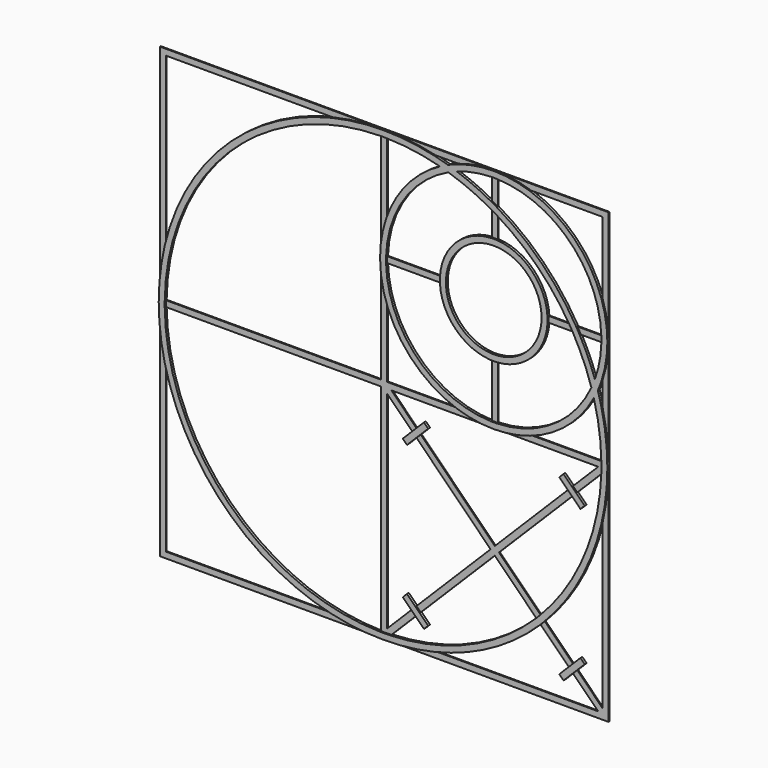
from build123d import *

# Parameters (mm, degrees)
F1_DEPTH = 0.8
F0_R     = 16
F2_DEPTH = 0.35


# Not quite as in the source:
# - a feature names something its author has since deleted; it is built from what else it names


with BuildPart() as f1:
    # F0 (on Front) → F1 (new body)
    with BuildSketch(Plane.XZ):
        with BuildLine():
            ThreePointArc((17.2103480163, 73.0397421615), (8.6659515201, 74.5380642902), (0.0056974823, 75.0397421615))
            ThreePointArc((0.0056974823, 75.0397421615), (-8.6545565556, 74.5380642902), (-17.1989530518, 73.0397421615))
            Line((-17.1989530518, 73.0397421615), (-0.9943025177, 73.0397421615))
            Line((-0.9943025177, 73.0397421615), (-0.9943025177, 73.032892525))
            ThreePointArc((-0.9943025177, 73.032892525), (0.0056974823, 73.0397421615), (1.0056974823, 73.032892525))
            Line((1.0056974823, 73.032892525), (1.0056974823, 73.0397421615))
            Line((1.0056974823, 73.0397421615), (17.2103480163, 73.0397421615))
        make_face()
        with BuildLine():
            ThreePointArc((-72.9943025177, 17.2443926956), (-74.4926246489, 8.6999961786), (-74.9943025177, 0.0397421197))
            ThreePointArc((-74.9943025177, 0.0397421197), (-74.4926246441, -8.6205118971), (-72.9943025177, -17.1649083727))
            Line((-72.9943025177, -17.1649083727), (-72.9943025177, -0.9602578386))
            Line((-72.9943025177, -0.9602578386), (-72.9874528813, -0.9602578386))
            ThreePointArc((-72.9874528813, -0.9602578386), (-72.9943025177, 0.0397421614), (-72.9874528813, 1.0397421615))
            Line((-72.9874528813, 1.0397421615), (-72.9943025177, 1.0397421615))
            Line((-72.9943025177, 1.0397421615), (-72.9943025177, 17.2443926956))
        make_face()
        with BuildLine():
            ThreePointArc((49.1712225429, 73.0397421615), (43.1701114913, 74.536408679), (37.0056974946, 75.0397421615))
            ThreePointArc((37.0056974946, 75.0397421615), (30.8412834854, 74.536408681), (24.8401724217, 73.0397421615))
            Line((24.8401724217, 73.0397421615), (36.0056974823, 73.0397421615))
            Line((36.0056974823, 73.0397421615), (37.0056974823, 73.0397421615))
            Line((37.0056974823, 73.0397421615), (38.0056974823, 73.0397421615))
            Line((38.0056974823, 73.0397421615), (49.1712225429, 73.0397421615))
        make_face()
        with BuildLine():
            ThreePointArc((21.7169774671, 71.8284621767), (19.4730859008, 72.4691615169), (17.2103480163, 73.0397421615))
            Line((17.2103480163, 73.0397421615), (1.0056974823, 73.0397421615))
            Line((1.0056974823, 73.0397421615), (1.0056974823, 73.032892525))
            ThreePointArc((1.0056974823, 73.032892525), (10.0952946195, 72.3391199569), (19.0275514161, 70.5178882276))
            ThreePointArc((19.0275514161, 70.5178882276), (20.3593616771, 71.199652938), (21.7169774671, 71.8284621767))
        make_face()
        with BuildLine():
            Line((-0.9943025177, 73.0397421615), (-17.1989530518, 73.0397421615))
            ThreePointArc((-17.1989530518, 73.0397421615), (-53.0273111067, 53.0727507504), (-72.9943025177, 17.2443926956))
            Line((-72.9943025177, 17.2443926956), (-72.9943025177, 1.0397421615))
            Line((-72.9943025177, 1.0397421615), (-72.9874528813, 1.0397421615))
            ThreePointArc((-72.9874528813, 1.0397421615), (-51.6130975444, 51.6585371881), (-0.9943025177, 73.032892525))
            Line((-0.9943025177, 73.032892525), (-0.9943025177, 73.0397421615))
        make_face()
        with BuildLine():
            Line((-72.9943025177, -0.9602578386), (-72.9943025177, -17.1649083727))
            ThreePointArc((-72.9943025177, -17.1649083727), (-53.0273111067, -52.9932664275), (-17.1989530518, -72.9602578385))
            Line((-17.1989530518, -72.9602578385), (-0.9943025177, -72.9602578385))
            Line((-0.9943025177, -72.9602578385), (-0.9943025177, -72.9534082021))
            ThreePointArc((-0.9943025177, -72.9534082021), (-51.6130975444, -51.5790528652), (-72.9874528813, -0.9602578386))
            Line((-72.9874528813, -0.9602578386), (-72.9943025177, -0.9602578386))
        make_face()
        with BuildLine():
            ThreePointArc((73.0056974823, 49.205267222), (63.8757551674, 63.9097998465), (49.1712225429, 73.0397421615))
            Line((49.1712225429, 73.0397421615), (38.0056974823, 73.0397421615))
            Line((38.0056974823, 73.0397421615), (38.0056974823, 73.0258505923))
            ThreePointArc((38.0056974823, 73.0258505923), (62.461541605, 62.4955862842), (72.9918059132, 38.0397421615))
            Line((72.9918059132, 38.0397421615), (73.0056974823, 38.0397421615))
            Line((73.0056974823, 38.0397421615), (73.0056974823, 49.205267222))
        make_face()
        with BuildLine():
            Line((36.0056974823, 73.0397421615), (24.8401724217, 73.0397421615))
            ThreePointArc((24.8401724217, 73.0397421615), (23.265221036, 72.4685342242), (21.7169774671, 71.8284621767))
            ThreePointArc((21.7169774671, 71.8284621767), (23.204042899, 71.3618058579), (24.6810902267, 70.864349417))
            ThreePointArc((24.6810902267, 70.864349417), (30.2563040679, 72.4013836468), (36.0056974823, 73.0258505923))
            Line((36.0056974823, 73.0258505923), (36.0056974823, 73.0397421615))
        make_face()
        with BuildLine():
            ThreePointArc((24.6810902267, 70.864349417), (23.204042899, 71.3618058579), (21.7169774671, 71.8284621767))
            ThreePointArc((21.7169774671, 71.8284621767), (20.3593616771, 71.199652938), (19.0275514161, 70.5178882276))
            ThreePointArc((19.0275514161, 70.5178882276), (20.4433919435, 70.1204145691), (21.8509385418, 69.6945011019))
            ThreePointArc((21.8509385418, 69.6945011019), (23.2535693595, 70.3095328445), (24.6810902267, 70.864349417))
        make_face()
        with BuildLine():
            ThreePointArc((-17.1989530518, -72.9602578385), (-8.6545565556, -74.4585799673), (0.0056974823, -74.9602578385))
            ThreePointArc((0.0056974823, -74.9602578385), (8.6659515201, -74.4585799673), (17.2103480163, -72.9602578386))
            Line((17.2103480163, -72.9602578385), (2.4199110446, -72.9602578385))
            Line((2.4199110446, -72.9602578385), (2.3812484608, -72.9215952547))
            ThreePointArc((2.3812484608, -72.9215952547), (0.6936568848, -72.957016067), (-0.9943025177, -72.9534082021))
            Line((-0.9943025177, -72.9534082021), (-0.9943025177, -72.9602578385))
            Line((-0.9943025177, -72.9602578385), (-17.1989530518, -72.9602578385))
        make_face()
        with BuildLine():
            ThreePointArc((73.0056974823, 24.8742171009), (74.5023640008, 30.8753281585), (75.0056974823, 37.0397421615))
            ThreePointArc((75.0056974823, 37.0397421615), (74.5023640008, 43.2041561644), (73.0056974823, 49.205267222))
            Line((73.0056974823, 49.205267222), (73.0056974823, 38.0397421615))
            Line((73.0056974823, 38.0397421615), (73.0056974823, 37.0397421615))
            Line((73.0056974823, 37.0397421615), (73.0056974823, 36.0397421615))
            Line((73.0056974823, 36.0397421615), (73.0056974823, 24.8742171009))
        make_face()
        with BuildLine():
            ThreePointArc((21.8509385418, 69.6945011019), (20.4433919435, 70.1204145691), (19.0275514161, 70.5178882276))
            ThreePointArc((19.0275514161, 70.5178882276), (7.9890295703, 61.5761025942), (1.0056974823, 49.205267222))
            Line((1.0056974823, 49.205267222), (1.0056974823, 38.0397421615))
            Line((1.0056974823, 38.0397421615), (1.0195890514, 38.0397421615))
            ThreePointArc((1.0195890514, 38.0397421614), (6.9332346671, 56.8298149312), (21.8509385418, 69.6945011019))
        make_face()
        with BuildLine():
            ThreePointArc((36.0056974823, 65.8348787598), (30.4474404505, 68.5838905992), (24.6810902267, 70.864349417))
            ThreePointArc((24.6810902267, 70.864349417), (23.2535693595, 70.3095328445), (21.8509385418, 69.6945011019))
            ThreePointArc((21.8509385418, 69.6945011019), (29.0912622658, 66.9951745118), (36.0056974823, 63.5456473987))
            Line((36.0056974823, 63.5456473987), (36.0056974823, 65.8348787598))
        make_face()
        with BuildLine():
            Line((2.4199110446, -72.9602578385), (17.2103480163, -72.9602578385))
            ThreePointArc((17.2103480163, -72.9602578386), (36.078425865, -65.7155486297), (52.3268850353, -53.695658954))
            Line((52.3268850353, -53.695658954), (50.9125423033, -52.281316222))
            ThreePointArc((50.9125423033, -52.281316222), (28.6127517607, -67.1215297556), (2.4612213459, -72.9189475373))
            Line((2.4612213459, -72.9189475373), (2.4199110446, -72.9602578385))
        make_face()
        with BuildLine():
            ThreePointArc((73.0056974823, -17.1649083726), (74.504019611, -8.6205118764), (75.0056974823, 0.0397421615))
            ThreePointArc((75.0056974823, 0.0397421615), (74.504019611, 8.6999961993), (73.0056974823, 17.2443926955))
            Line((73.0056974823, 17.2443926955), (73.0056974823, 1.0397421615))
            Line((73.0056974823, 1.0397421615), (72.9988478458, 1.0397421615))
            ThreePointArc((72.9988478458, 1.0397421615), (73.0039850531, 0.5397538907), (73.0056974823, 0.0397421615))
            ThreePointArc((73.0056974823, 0.0397421615), (72.9960311963, -1.1481906278), (72.9670348984, -2.335808817))
            Line((72.9670348984, -2.335808817), (73.0056974823, -2.3744714009))
            Line((73.0056974823, -2.3744714009), (73.0056974823, -17.1649083726))
        make_face()
        with BuildLine():
            ThreePointArc((71.7944174975, 21.7510221462), (72.4344895451, 23.2992657152), (73.0056974823, 24.8742171009))
            Line((73.0056974823, 24.8742171009), (73.0056974823, 36.0397421615))
            Line((73.0056974823, 36.0397421615), (72.9918059132, 36.0397421615))
            ThreePointArc((72.9918059132, 36.0397421615), (72.3673389676, 30.2903487471), (70.8303047379, 24.7151349058))
            ThreePointArc((70.8303047379, 24.7151349058), (71.3277611788, 23.2380875782), (71.7944174975, 21.7510221462))
        make_face()
        with BuildLine():
            Line((1.0056974823, 38.0397421615), (1.0056974823, 49.205267222))
            ThreePointArc((1.0056974823, 49.205267222), (-0.4909690583, 43.20415603), (-0.9943025177, 37.0397418891))
            ThreePointArc((-0.9943025177, 37.0397418891), (-0.4909690141, 30.8753280241), (1.0056974823, 24.8742171009))
            Line((1.0056974823, 24.8742171009), (1.0056974823, 36.0397421615))
            Line((1.0056974823, 36.0397421615), (1.0056974823, 37.0397421615))
            Line((1.0056974823, 37.0397421615), (1.0056974823, 38.0397421615))
        make_face()
        with BuildLine():
            ThreePointArc((38.0056974823, 64.7003948028), (37.0100453817, 65.2753017631), (36.0056974823, 65.8348787598))
            Line((36.0056974823, 65.8348787598), (36.0056974823, 63.5456473987))
            ThreePointArc((36.0056974823, 63.5456473987), (37.0103704926, 62.9655252348), (38.0056974823, 62.3695103304))
            Line((38.0056974823, 62.3695103304), (38.0056974823, 64.7003948028))
        make_face()
        with BuildLine():
            Line((50.9125423033, -52.281316222), (52.3268850353, -53.695658954))
            ThreePointArc((52.3268850353, -53.695658954), (53.0387060713, -52.9932664275), (53.7410985977, -52.2814453916))
            Line((53.7410985977, -52.2814453916), (52.3267558657, -50.8671026596))
            ThreePointArc((52.3267558657, -50.8671026596), (51.6244925089, -51.5790528652), (50.9125423033, -52.281316222))
        make_face()
        with BuildLine():
            Line((73.0056974823, 1.0397421615), (73.0056974823, 17.2443926955))
            ThreePointArc((73.0056974823, 17.2443926955), (72.4351168377, 19.50713058), (71.7944174975, 21.7510221462))
            ThreePointArc((71.7944174975, 21.7510221462), (71.1656082588, 20.3934063563), (70.4838435484, 19.0615960953))
            ThreePointArc((70.4838435484, 19.0615960953), (72.3050752777, 10.1293392987), (72.9988478458, 1.0397421615))
            Line((72.9988478458, 1.0397421615), (73.0056974823, 1.0397421615))
        make_face()
        with BuildLine():
            ThreePointArc((53.7410985977, -52.2814453916), (65.7609882734, -36.0329862213), (73.0056974823, -17.1649083726))
            Line((73.0056974823, -17.1649083726), (73.0056974823, -2.3744714009))
            Line((73.0056974823, -2.3744714009), (72.964387181, -2.4157817022))
            ThreePointArc((72.964387181, -2.4157817022), (67.1669693993, -28.5673121169), (52.3267558657, -50.8671026596))
            Line((52.3267558657, -50.8671026596), (53.7410985977, -52.2814453916))
        make_face()
        with BuildLine():
            ThreePointArc((70.4838435484, 19.0615960953), (71.1656082588, 20.3934063563), (71.7944174975, 21.7510221462))
            ThreePointArc((71.7944174975, 21.7510221462), (71.3277611788, 23.2380875782), (70.8303047379, 24.7151349058))
            ThreePointArc((70.8303047379, 24.7151349058), (70.2754881653, 23.2876140387), (69.6604564227, 21.884983221))
            ThreePointArc((69.6604564227, 21.884983221), (70.0863698899, 20.4774366227), (70.4838435484, 19.0615960953))
        make_face()
        with BuildLine():
            ThreePointArc((64.6663501236, 38.0397421615), (53.0387060713, 53.0727507504), (38.0056974823, 64.7003948028))
            Line((38.0056974823, 64.7003948028), (38.0056974823, 62.3695103304))
            ThreePointArc((38.0056974823, 62.3695103304), (51.6244925089, 51.6585371881), (62.3354656513, 38.0397421615))
            Line((62.3354656513, 38.0397421615), (64.6663501236, 38.0397421615))
        make_face()
        with BuildLine():
            Line((1.0056974823, 36.0397421615), (1.0056974823, 24.8742171009))
            ThreePointArc((1.0056974823, 24.8742171009), (10.1356397972, 10.1696844764), (24.8401724217, 1.0397421615))
            Line((24.8401724217, 1.0397421615), (36.0056974823, 1.0397421615))
            Line((36.0056974823, 1.0397421615), (36.0056974823, 1.0536337306))
            ThreePointArc((36.0056974823, 1.0536337306), (11.5498533596, 11.5838980387), (1.0195890514, 36.0397421615))
            Line((1.0195890514, 36.0397421615), (1.0056974823, 36.0397421615))
        make_face()
        with BuildLine():
            ThreePointArc((49.1712225429, 1.0397421615), (61.542057915, 8.0230742494), (70.4838435484, 19.0615960953))
            ThreePointArc((70.4838435484, 19.0615960953), (70.0863698899, 20.4774366227), (69.6604564227, 21.884983221))
            ThreePointArc((69.6604564227, 21.884983221), (56.795770252, 6.9672793463), (38.0056974823, 1.0536337306))
            Line((38.0056974823, 1.0536337306), (38.0056974823, 1.0397421615))
            Line((38.0056974823, 1.0397421615), (49.1712225429, 1.0397421615))
        make_face()
        with BuildLine():
            ThreePointArc((69.6604564227, 21.884983221), (70.2754881653, 23.2876140387), (70.8303047379, 24.7151349058))
            ThreePointArc((70.8303047379, 24.7151349058), (68.54984592, 30.4814851297), (65.8008340806, 36.0397421615))
            Line((65.8008340806, 36.0397421615), (63.5116027195, 36.0397421615))
            ThreePointArc((63.5116027195, 36.0397421615), (66.9611298326, 29.125306945), (69.6604564227, 21.884983221))
        make_face()
        with BuildLine():
            ThreePointArc((65.8008340806, 36.0397421615), (65.2412570839, 37.0440900609), (64.6663501236, 38.0397421615))
            Line((64.6663501236, 38.0397421615), (62.3354656513, 38.0397421615))
            ThreePointArc((62.3354656513, 38.0397421615), (62.9314805557, 37.0444151718), (63.5116027195, 36.0397421615))
            Line((63.5116027195, 36.0397421615), (65.8008340806, 36.0397421615))
        make_face()
        with BuildLine():
            Line((36.0056974823, 1.0397421615), (24.8401724217, 1.0397421615))
            ThreePointArc((24.8401724217, 1.0397421615), (30.8412834793, -0.4569243571), (37.0056974823, -0.9602578385))
            ThreePointArc((37.0056974823, -0.9602578385), (43.1701114852, -0.4569243571), (49.1712225429, 1.0397421615))
            Line((49.1712225429, 1.0397421615), (38.0056974823, 1.0397421615))
            Line((38.0056974823, 1.0397421615), (37.0056976148, 1.0397421615))
            Line((37.0056976148, 1.0397421615), (36.0056974823, 1.0397421615))
        make_face()
    extrude(amount=F1_DEPTH)


with BuildPart() as f1b:
    # F0 (on Front) → F1, piece 2 (new body)
    with BuildSketch(Plane.XZ):
        Polygon((60.3402212614, -67.3658494296), (63.1686483862, -64.5374223048), (61.7544348238, -63.1232087424), (58.9260076991, -65.9516358672), align=None)
        Polygon((61.7544348238, -63.1232087424), (63.1686483862, -64.5374223048), (64.5828619485, -63.1232087424), (63.1686483862, -61.7089951801), align=None)
        Polygon((63.1686483862, -61.7089951801), (64.5828619485, -63.1232087424), (67.4112890733, -60.2947816177), (65.9970755109, -58.8805680553), align=None)
    extrude(amount=F1_DEPTH)


with BuildPart() as f1c:
    # F0 (on Front) → F1, piece 3 (new body)
    with BuildSketch(Plane.XZ):
        with BuildLine():
            ThreePointArc((36.0056974823, 55.0119429171), (24.2777754209, 49.7676642228), (19.0334967267, 38.0397421615))
            ThreePointArc((19.0334967267, 38.0397421615), (19.0056974823, 37.0397421615), (19.0334967267, 36.0397421615))
            ThreePointArc((19.0334967267, 36.0397421615), (24.2777754209, 24.3118201001), (36.0056974823, 19.0675414058))
            ThreePointArc((36.0056974823, 19.0675414058), (37.0056974823, 19.0397421615), (38.0056974823, 19.0675414058))
            ThreePointArc((38.0056974823, 19.0675414058), (49.7336195436, 24.3118201001), (54.9778982379, 36.0397421615))
            ThreePointArc((54.9778982379, 36.0397421615), (54.998746329, 36.5395489993), (55.0056974823, 37.0397421615))
            ThreePointArc((55.0056974823, 37.0397421615), (54.998746329, 37.5399353236), (54.9778982379, 38.0397421615))
            ThreePointArc((54.9778982379, 38.0397421615), (49.7336195436, 49.7676642228), (38.0056974823, 55.0119429171))
            ThreePointArc((38.0056974823, 55.0119429171), (37.0056974823, 55.0397421615), (36.0056974823, 55.0119429171))
        make_face()
        with Locations((37.0056974823, 37.0397421615)):
            Circle(F0_R, mode=Mode.SUBTRACT)
    extrude(amount=F1_DEPTH)


with BuildPart() as f1d:
    # F0 (on Front) → F1, piece 4 (new body)
    with BuildSketch(Plane.XZ):
        Polygon((9.428533016, -63.1232087424), (10.8427465784, -64.5374223048), (12.2569601407, -63.1232087424), (10.8427465784, -61.7089951801), align=None)
        Polygon((12.2569601407, -63.1232087424), (10.8427465784, -64.5374223048), (13.6711737031, -67.3658494296), (15.0853872655, -65.9516358672), align=None)
        Polygon((6.6001058912, -60.2947816177), (9.428533016, -63.1232087424), (10.8427465784, -61.7089951801), (8.0143194536, -58.8805680553), align=None)
    extrude(amount=F1_DEPTH)


with BuildPart() as f1e:
    # F0 (on Front) → F1, piece 5 (new body)
    with BuildSketch(Plane.XZ):
        Polygon((67.4112890733, -13.6257340594), (64.5828619485, -10.7973069346), (63.1686483862, -12.211520497), (65.9970755109, -15.0399476218), align=None)
        Polygon((63.1686483862, -12.211520497), (64.5828619485, -10.7973069346), (63.1686483862, -9.3830933723), (61.7544348238, -10.7973069346), align=None)
        Polygon((61.7544348238, -10.7973069346), (63.1686483862, -9.3830933723), (60.3402212614, -6.5546662475), (58.9260076991, -7.9688798099), align=None)
    extrude(amount=F1_DEPTH)


with BuildPart() as f1f:
    # F0 (on Front) → F1, piece 6 (new body)
    with BuildSketch(Plane.XZ):
        Polygon((10.8427465784, -9.3830933723), (9.428533016, -10.7973069346), (10.8427465784, -12.211520497), (12.2569601407, -10.7973069346), align=None)
        Polygon((10.8427465784, -12.211520497), (9.428533016, -10.7973069346), (6.6001058912, -13.6257340594), (8.0143194536, -15.0399476218), align=None)
        Polygon((13.6711737031, -6.5546662475), (10.8427465784, -9.3830933723), (12.2569601407, -10.7973069346), (15.0853872655, -7.9688798099), align=None)
    extrude(amount=F1_DEPTH)


with BuildPart() as f2:
    # F0 (on Front) → F2 (new body)
    with BuildSketch(Plane.XZ):
        with BuildLine():
            ThreePointArc((17.2103480163, -72.9602578386), (8.6659515201, -74.4585799673), (0.0056974823, -74.9602578385))
            Line((0.0056974823, -74.9602578385), (75.0056974823, -74.9602578385))
            Line((75.0056974823, -74.9602578385), (75.0056974823, 0.0397421615))
            ThreePointArc((75.0056974823, 0.0397421615), (74.504019611, -8.6205118764), (73.0056974823, -17.1649083726))
            Line((73.0056974823, -17.1649083726), (73.0056974823, -71.5460442762))
            Line((73.0056974823, -71.5460442762), (71.5914839199, -72.9602578385))
            Line((71.5914839199, -72.9602578385), (17.2103480163, -72.9602578385))
        make_face()
        with BuildLine():
            Line((0.0056974823, 75.0397421615), (-74.9943025177, 75.0397421615))
            Line((-74.9943025177, 75.0397421615), (-74.9943025177, 0.0397421197))
            ThreePointArc((-74.9943025177, 0.0397421197), (-74.4926246489, 8.6999961786), (-72.9943025177, 17.2443926956))
            Line((-72.9943025177, 17.2443926956), (-72.9943025177, 73.0397421615))
            Line((-72.9943025177, 73.0397421615), (-17.1989530518, 73.0397421615))
            ThreePointArc((-17.1989530518, 73.0397421615), (-8.6545565556, 74.5380642902), (0.0056974823, 75.0397421615))
        make_face()
        Polygon((2.4199110446, -0.9602578385), (1.0056974823, -2.3744714009), (9.428533016, -10.7973069346), (10.8427465784, -9.3830933723), align=None)
        with BuildLine():
            Line((37.0056974823, -38.3744714009), (50.9125423033, -52.281316222))
            ThreePointArc((50.9125423033, -52.281316222), (51.6244925089, -51.5790528652), (52.3267558657, -50.8671026596))
            Line((52.3267558657, -50.8671026596), (38.4199110446, -36.9602578385))
            Line((38.4199110446, -36.9602578385), (63.1686483862, -12.211520497))
            Line((63.1686483862, -12.211520497), (61.7544348238, -10.7973069346))
            Line((61.7544348238, -10.7973069346), (37.0056974823, -35.5460442762))
            Line((37.0056974823, -35.5460442762), (12.2569601407, -10.7973069346))
            Line((12.2569601407, -10.7973069346), (10.8427465784, -12.211520497))
            Line((10.8427465784, -12.211520497), (35.5914839199, -36.9602578385))
            Line((35.5914839199, -36.9602578385), (10.8427465784, -61.7089951801))
            Line((10.8427465784, -61.7089951801), (12.2569601407, -63.1232087424))
            Line((12.2569601407, -63.1232087424), (37.0056974823, -38.3744714009))
        make_face()
        with BuildLine():
            Line((72.964387181, -2.4157817022), (73.0056974823, -2.3744714009))
            Line((73.0056974823, -2.3744714009), (72.9670348984, -2.335808817))
            ThreePointArc((72.9670348984, -2.335808817), (72.9657219972, -2.3757956224), (72.964387181, -2.4157817022))
        make_face()
        Polygon((63.1686483862, -64.5374223048), (71.5914839199, -72.9602578385), (73.0056974823, -71.5460442762), (64.5828619485, -63.1232087424), align=None)
        with BuildLine():
            Line((2.3812484608, -72.9215952547), (2.4199110446, -72.9602578385))
            Line((2.4199110446, -72.9602578385), (2.4612213459, -72.9189475373))
            ThreePointArc((2.4612213459, -72.9189475373), (2.4212352661, -72.9202823534), (2.3812484608, -72.9215952547))
        make_face()
        with BuildLine():
            ThreePointArc((53.7410985977, -52.2814453916), (53.0387060713, -52.9932664275), (52.3268850353, -53.695658954))
            Line((52.3268850353, -53.695658954), (61.7544348238, -63.1232087424))
            Line((61.7544348238, -63.1232087424), (63.1686483862, -61.7089951801))
            Line((63.1686483862, -61.7089951801), (53.7410985977, -52.2814453916))
        make_face()
        with BuildLine():
            Line((50.9125423033, -52.281316222), (52.3268850353, -53.695658954))
            ThreePointArc((52.3268850353, -53.695658954), (53.0387060713, -52.9932664275), (53.7410985977, -52.2814453916))
            Line((53.7410985977, -52.2814453916), (52.3267558657, -50.8671026596))
            ThreePointArc((52.3267558657, -50.8671026596), (51.6244925089, -51.5790528652), (50.9125423033, -52.281316222))
        make_face()
        with BuildLine():
            Line((37.0056974946, 75.0397421615), (0.0056974823, 75.0397421615))
            ThreePointArc((0.0056974823, 75.0397421615), (8.6659515201, 74.5380642902), (17.2103480163, 73.0397421615))
            Line((17.2103480163, 73.0397421615), (24.8401724217, 73.0397421615))
            ThreePointArc((24.8401724217, 73.0397421615), (30.8412834854, 74.536408681), (37.0056974946, 75.0397421615))
        make_face()
        with BuildLine():
            Line((75.0056974823, 75.0397421615), (37.0056974946, 75.0397421615))
            ThreePointArc((37.0056974946, 75.0397421615), (43.1701114913, 74.536408679), (49.1712225429, 73.0397421615))
            Line((49.1712225429, 73.0397421615), (73.0056974823, 73.0397421615))
            Line((73.0056974823, 73.0397421615), (73.0056974823, 49.205267222))
            ThreePointArc((73.0056974823, 49.205267222), (74.5023640008, 43.2041561644), (75.0056974823, 37.0397421615))
            Line((75.0056974823, 37.0397421615), (75.0056974823, 75.0397421615))
        make_face()
        with BuildLine():
            Line((75.0056974823, 0.0397421615), (75.0056974823, 37.0397421615))
            ThreePointArc((75.0056974823, 37.0397421615), (74.5023640008, 30.8753281585), (73.0056974823, 24.8742171009))
            Line((73.0056974823, 24.8742171009), (73.0056974823, 17.2443926955))
            ThreePointArc((73.0056974823, 17.2443926955), (74.504019611, 8.6999961993), (75.0056974823, 0.0397421615))
        make_face()
        with BuildLine():
            ThreePointArc((73.0056974823, -17.1649083726), (74.504019611, -8.6205118764), (75.0056974823, 0.0397421615))
            ThreePointArc((75.0056974823, 0.0397421615), (74.504019611, 8.6999961993), (73.0056974823, 17.2443926955))
            Line((73.0056974823, 17.2443926955), (73.0056974823, 1.0397421615))
            Line((73.0056974823, 1.0397421615), (72.9988478458, 1.0397421615))
            ThreePointArc((72.9988478458, 1.0397421615), (73.0039850531, 0.5397538907), (73.0056974823, 0.0397421615))
            ThreePointArc((73.0056974823, 0.0397421615), (72.9960311963, -1.1481906278), (72.9670348984, -2.335808817))
            Line((72.9670348984, -2.335808817), (73.0056974823, -2.3744714009))
            Line((73.0056974823, -2.3744714009), (73.0056974823, -17.1649083726))
        make_face()
        with BuildLine():
            ThreePointArc((73.0056974823, 24.8742171009), (74.5023640008, 30.8753281585), (75.0056974823, 37.0397421615))
            ThreePointArc((75.0056974823, 37.0397421615), (74.5023640008, 43.2041561644), (73.0056974823, 49.205267222))
            Line((73.0056974823, 49.205267222), (73.0056974823, 38.0397421615))
            Line((73.0056974823, 38.0397421615), (73.0056974823, 37.0397421615))
            Line((73.0056974823, 37.0397421615), (73.0056974823, 36.0397421615))
            Line((73.0056974823, 36.0397421615), (73.0056974823, 24.8742171009))
        make_face()
        with BuildLine():
            ThreePointArc((49.1712225429, 73.0397421615), (43.1701114913, 74.536408679), (37.0056974946, 75.0397421615))
            ThreePointArc((37.0056974946, 75.0397421615), (30.8412834854, 74.536408681), (24.8401724217, 73.0397421615))
            Line((24.8401724217, 73.0397421615), (36.0056974823, 73.0397421615))
            Line((36.0056974823, 73.0397421615), (37.0056974823, 73.0397421615))
            Line((37.0056974823, 73.0397421615), (38.0056974823, 73.0397421615))
            Line((38.0056974823, 73.0397421615), (49.1712225429, 73.0397421615))
        make_face()
        with BuildLine():
            ThreePointArc((17.2103480163, 73.0397421615), (8.6659515201, 74.5380642902), (0.0056974823, 75.0397421615))
            ThreePointArc((0.0056974823, 75.0397421615), (-8.6545565556, 74.5380642902), (-17.1989530518, 73.0397421615))
            Line((-17.1989530518, 73.0397421615), (-0.9943025177, 73.0397421615))
            Line((-0.9943025177, 73.0397421615), (-0.9943025177, 73.032892525))
            ThreePointArc((-0.9943025177, 73.032892525), (0.0056974823, 73.0397421615), (1.0056974823, 73.032892525))
            Line((1.0056974823, 73.032892525), (1.0056974823, 73.0397421615))
            Line((1.0056974823, 73.0397421615), (17.2103480163, 73.0397421615))
        make_face()
        with BuildLine():
            Line((1.0056974823, 49.205267222), (1.0056974823, 73.032892525))
            ThreePointArc((1.0056974823, 73.032892525), (0.0056974823, 73.0397421615), (-0.9943025177, 73.032892525))
            Line((-0.9943025177, 73.032892525), (-0.9943025177, 37.0397418891))
            ThreePointArc((-0.9943025177, 37.0397418891), (-0.4909690583, 43.20415603), (1.0056974823, 49.205267222))
        make_face()
        with BuildLine():
            Line((1.0056974823, 38.0397421615), (1.0056974823, 49.205267222))
            ThreePointArc((1.0056974823, 49.205267222), (-0.4909690583, 43.20415603), (-0.9943025177, 37.0397418891))
            ThreePointArc((-0.9943025177, 37.0397418891), (-0.4909690141, 30.8753280241), (1.0056974823, 24.8742171009))
            Line((1.0056974823, 24.8742171009), (1.0056974823, 36.0397421615))
            Line((1.0056974823, 36.0397421615), (1.0056974823, 37.0397421615))
            Line((1.0056974823, 37.0397421615), (1.0056974823, 38.0397421615))
        make_face()
        with BuildLine():
            Line((-0.9943025177, 1.0397421615), (-72.9874528813, 1.0397421615))
            ThreePointArc((-72.9874528813, 1.0397421615), (-72.9943025177, 0.0397421614), (-72.9874528813, -0.9602578386))
            Line((-72.9874528813, -0.9602578386), (-0.9943025177, -0.9602578385))
            Line((-0.9943025177, -0.9602578385), (-0.9943025177, -72.9534082021))
            ThreePointArc((-0.9943025177, -72.9534082021), (0.6936568848, -72.957016067), (2.3812484608, -72.9215952547))
            Line((2.3812484608, -72.9215952547), (1.0056974823, -71.5460442762))
            Line((1.0056974823, -71.5460442762), (1.0056974823, -2.3744714009))
            Line((1.0056974823, -2.3744714009), (2.4199110446, -0.9602578385))
            Line((2.4199110446, -0.9602578385), (37.0056974823, -0.9602578385))
            ThreePointArc((37.0056974823, -0.9602578385), (30.8412834793, -0.4569243571), (24.8401724217, 1.0397421615))
            Line((24.8401724217, 1.0397421615), (1.0056974823, 1.0397421615))
            Line((1.0056974823, 1.0397421615), (1.0056974823, 24.8742171009))
            ThreePointArc((1.0056974823, 24.8742171009), (-0.4909690141, 30.8753280241), (-0.9943025177, 37.0397418891))
            Line((-0.9943025177, 37.0397418891), (-0.9943025177, 1.0397421615))
        make_face()
        with BuildLine():
            ThreePointArc((-72.9943025177, -17.1649083727), (-74.4926246441, -8.6205118971), (-74.9943025177, 0.0397421197))
            Line((-74.9943025177, 0.0397421197), (-74.9943025177, -74.9602578385))
            Line((-74.9943025177, -74.9602578385), (0.0056974823, -74.9602578385))
            ThreePointArc((0.0056974823, -74.9602578385), (-8.6545565556, -74.4585799673), (-17.1989530518, -72.9602578385))
            Line((-17.1989530518, -72.9602578385), (-72.9943025177, -72.9602578385))
            Line((-72.9943025177, -72.9602578385), (-72.9943025177, -17.1649083727))
        make_face()
        with BuildLine():
            ThreePointArc((-72.9943025177, 17.2443926956), (-74.4926246489, 8.6999961786), (-74.9943025177, 0.0397421197))
            ThreePointArc((-74.9943025177, 0.0397421197), (-74.4926246441, -8.6205118971), (-72.9943025177, -17.1649083727))
            Line((-72.9943025177, -17.1649083727), (-72.9943025177, -0.9602578386))
            Line((-72.9943025177, -0.9602578386), (-72.9874528813, -0.9602578386))
            ThreePointArc((-72.9874528813, -0.9602578386), (-72.9943025177, 0.0397421614), (-72.9874528813, 1.0397421615))
            Line((-72.9874528813, 1.0397421615), (-72.9943025177, 1.0397421615))
            Line((-72.9943025177, 1.0397421615), (-72.9943025177, 17.2443926956))
        make_face()
        with BuildLine():
            ThreePointArc((-17.1989530518, -72.9602578385), (-8.6545565556, -74.4585799673), (0.0056974823, -74.9602578385))
            ThreePointArc((0.0056974823, -74.9602578385), (8.6659515201, -74.4585799673), (17.2103480163, -72.9602578386))
            Line((17.2103480163, -72.9602578385), (2.4199110446, -72.9602578385))
            Line((2.4199110446, -72.9602578385), (2.3812484608, -72.9215952547))
            ThreePointArc((2.3812484608, -72.9215952547), (0.6936568848, -72.957016067), (-0.9943025177, -72.9534082021))
            Line((-0.9943025177, -72.9534082021), (-0.9943025177, -72.9602578385))
            Line((-0.9943025177, -72.9602578385), (-17.1989530518, -72.9602578385))
        make_face()
        with BuildLine():
            ThreePointArc((2.3812484608, -72.9215952547), (2.4212352661, -72.9202823534), (2.4612213459, -72.9189475373))
            Line((2.4612213459, -72.9189475373), (10.8427465784, -64.5374223048))
            Line((10.8427465784, -64.5374223048), (9.428533016, -63.1232087424))
            Line((9.428533016, -63.1232087424), (1.0056974823, -71.5460442762))
            Line((1.0056974823, -71.5460442762), (2.3812484608, -72.9215952547))
        make_face()
        Polygon((9.428533016, -63.1232087424), (10.8427465784, -64.5374223048), (12.2569601407, -63.1232087424), (10.8427465784, -61.7089951801), align=None)
        Polygon((61.7544348238, -63.1232087424), (63.1686483862, -64.5374223048), (64.5828619485, -63.1232087424), (63.1686483862, -61.7089951801), align=None)
        Polygon((63.1686483862, -12.211520497), (64.5828619485, -10.7973069346), (63.1686483862, -9.3830933723), (61.7544348238, -10.7973069346), align=None)
        with BuildLine():
            Line((64.5828619485, -10.7973069346), (72.964387181, -2.4157817022))
            ThreePointArc((72.964387181, -2.4157817022), (72.9657219972, -2.3757956224), (72.9670348984, -2.335808817))
            Line((72.9670348984, -2.335808817), (71.5914839199, -0.9602578385))
            Line((71.5914839199, -0.9602578385), (63.1686483862, -9.3830933723))
            Line((63.1686483862, -9.3830933723), (64.5828619485, -10.7973069346))
        make_face()
        with BuildLine():
            ThreePointArc((73.0056974823, 0.0397421615), (73.0039850531, 0.5397538907), (72.9988478458, 1.0397421615))
            Line((72.9988478458, 1.0397421615), (49.1712225429, 1.0397421615))
            ThreePointArc((49.1712225429, 1.0397421615), (43.1701114852, -0.4569243571), (37.0056974823, -0.9602578385))
            Line((37.0056974823, -0.9602578385), (71.5914839199, -0.9602578385))
            Line((71.5914839199, -0.9602578385), (72.9670348984, -2.335808817))
            ThreePointArc((72.9670348984, -2.335808817), (72.9960311963, -1.1481906278), (73.0056974823, 0.0397421615))
        make_face()
        with BuildLine():
            Line((36.0056974823, 1.0397421615), (24.8401724217, 1.0397421615))
            ThreePointArc((24.8401724217, 1.0397421615), (30.8412834793, -0.4569243571), (37.0056974823, -0.9602578385))
            ThreePointArc((37.0056974823, -0.9602578385), (43.1701114852, -0.4569243571), (49.1712225429, 1.0397421615))
            Line((49.1712225429, 1.0397421615), (38.0056974823, 1.0397421615))
            Line((38.0056974823, 1.0397421615), (37.0056976148, 1.0397421615))
            Line((37.0056976148, 1.0397421615), (36.0056974823, 1.0397421615))
        make_face()
        Polygon((10.8427465784, -9.3830933723), (9.428533016, -10.7973069346), (10.8427465784, -12.211520497), (12.2569601407, -10.7973069346), align=None)
    extrude(amount=F2_DEPTH)


with BuildPart() as f2b:
    # F0 (on Front) → F2, piece 2 (new body)
    with BuildSketch(Plane.XZ):
        with BuildLine():
            Line((19.0334967267, 38.0397421615), (1.0195890514, 38.0397421615))
            ThreePointArc((1.0195890514, 38.0397421614), (1.0091705421, 37.539790403), (1.0056974823, 37.0397421615))
            ThreePointArc((1.0056974823, 37.0397421615), (1.0091705421, 36.5396939199), (1.0195890514, 36.0397421615))
            Line((1.0195890514, 36.0397421615), (19.0334967267, 36.0397421615))
            ThreePointArc((19.0334967267, 36.0397421615), (19.0056974823, 37.0397421615), (19.0334967267, 38.0397421615))
        make_face()
    extrude(amount=F2_DEPTH)


with BuildPart() as f2c:
    # F0 (on Front) → F2, piece 3 (new body)
    with BuildSketch(Plane.XZ):
        with BuildLine():
            ThreePointArc((37.0056976148, 1.0397421615), (37.5057457901, 1.0432152222), (38.0056974823, 1.0536337306))
            Line((38.0056974823, 1.0536337306), (38.0056974823, 19.0675414058))
            ThreePointArc((38.0056974823, 19.0675414058), (37.0056974823, 19.0397421615), (36.0056974823, 19.0675414058))
            Line((36.0056974823, 19.0675414058), (36.0056974823, 1.0536337306))
            ThreePointArc((36.0056974823, 1.0536337306), (36.5056493069, 1.0432152203), (37.0056976148, 1.0397421615))
        make_face()
    extrude(amount=F2_DEPTH)


with BuildPart() as f2d:
    # F0 (on Front) → F2, piece 4 (new body)
    with BuildSketch(Plane.XZ):
        with BuildLine():
            Line((38.0056974823, 64.7003948028), (38.0056974823, 73.0258505923))
            ThreePointArc((38.0056974823, 73.0258505923), (37.5057457239, 73.0362691016), (37.0056974823, 73.0397421615))
            ThreePointArc((37.0056974823, 73.0397421615), (36.5056492407, 73.0362691016), (36.0056974823, 73.0258505923))
            Line((36.0056974823, 73.0258505923), (36.0056974823, 65.8348787598))
            ThreePointArc((36.0056974823, 65.8348787598), (37.0100453817, 65.2753017631), (38.0056974823, 64.7003948028))
        make_face()
        with BuildLine():
            ThreePointArc((38.0056974823, 64.7003948028), (37.0100453817, 65.2753017631), (36.0056974823, 65.8348787598))
            Line((36.0056974823, 65.8348787598), (36.0056974823, 63.5456473987))
            ThreePointArc((36.0056974823, 63.5456473987), (37.0103704926, 62.9655252348), (38.0056974823, 62.3695103304))
            Line((38.0056974823, 62.3695103304), (38.0056974823, 64.7003948028))
        make_face()
        with BuildLine():
            ThreePointArc((38.0056974823, 62.3695103304), (37.0103704926, 62.9655252348), (36.0056974823, 63.5456473987))
            Line((36.0056974823, 63.5456473987), (36.0056974823, 55.0119429171))
            ThreePointArc((36.0056974823, 55.0119429171), (37.0056974823, 55.0397421615), (38.0056974823, 55.0119429171))
            Line((38.0056974823, 55.0119429171), (38.0056974823, 62.3695103304))
        make_face()
    extrude(amount=F2_DEPTH)


with BuildPart() as f2e:
    # F0 (on Front) → F2, piece 5 (new body)
    with BuildSketch(Plane.XZ):
        with BuildLine():
            ThreePointArc((73.0056974823, 37.0397421615), (73.0022244225, 37.539790403), (72.9918059132, 38.0397421615))
            Line((72.9918059132, 38.0397421615), (64.6663501236, 38.0397421615))
            ThreePointArc((64.6663501236, 38.0397421615), (65.2412570839, 37.0440900609), (65.8008340806, 36.0397421615))
            Line((65.8008340806, 36.0397421615), (72.9918059132, 36.0397421615))
            ThreePointArc((72.9918059132, 36.0397421615), (73.0022244225, 36.5396939199), (73.0056974823, 37.0397421615))
        make_face()
        with BuildLine():
            ThreePointArc((63.5116027195, 36.0397421615), (62.9314805557, 37.0444151718), (62.3354656513, 38.0397421615))
            Line((62.3354656513, 38.0397421615), (54.9778982379, 38.0397421615))
            ThreePointArc((54.9778982379, 38.0397421615), (54.998746329, 37.5399353236), (55.0056974823, 37.0397421615))
            ThreePointArc((55.0056974823, 37.0397421615), (54.998746329, 36.5395489993), (54.9778982379, 36.0397421615))
            Line((54.9778982379, 36.0397421615), (63.5116027195, 36.0397421615))
        make_face()
        with BuildLine():
            ThreePointArc((65.8008340806, 36.0397421615), (65.2412570839, 37.0440900609), (64.6663501236, 38.0397421615))
            Line((64.6663501236, 38.0397421615), (62.3354656513, 38.0397421615))
            ThreePointArc((62.3354656513, 38.0397421615), (62.9314805557, 37.0444151718), (63.5116027195, 36.0397421615))
            Line((63.5116027195, 36.0397421615), (65.8008340806, 36.0397421615))
        make_face()
    extrude(amount=F2_DEPTH)


solid = Compound([f1.part, f1b.part, f1c.part, f1d.part, f1e.part, f1f.part, f2.part, f2b.part, f2c.part, f2d.part, f2e.part])
